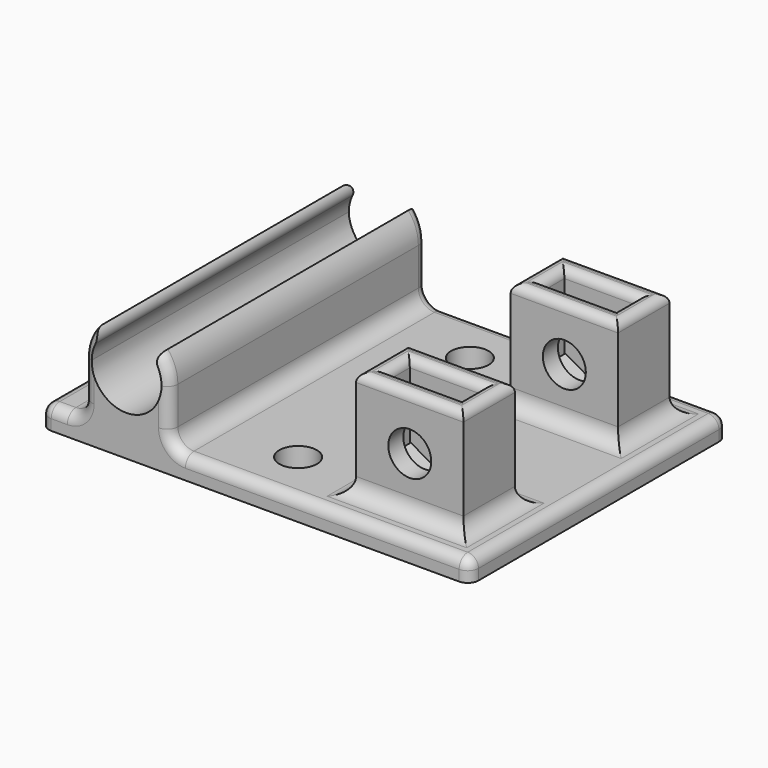
from build123d import *

# Parameters (mm, degrees)
F0_W          = 40
F0_H          = 30
F0_R          = 1.75
F1_DEPTH      = 2
F0_W_2        = 6.8
F0_H_2        = 2.5
F0_W_3        = 10
F0_H_3        = 6
F0_H_4        = 12
F2_DEPTH      = 12
F3_R          = 2
F4_DEPTH      = 24
F5_DEPTH      = 24
F6_START      = 2
F6_DEPTH      = 10
F7_R          = 1.5
F8_R          = 0.79999
F11_DEPTH     = 30
F12_T1_DEPTH  = 33.8160542738
F13_R         = 1.5
F14_T1_DEPTH  = 3.5
F14_T3_DEPTH  = 28
F14_T5_DEPTH  = 1.5
F14_T7_DEPTH  = 25.5
F14_T9_DEPTH  = 3.5
F14_S13_W     = 1
F14_S13_H     = 1
F14_T14_DEPTH = 1
F14_S19_W     = 1
F14_S19_H     = 1
F14_T20_DEPTH = 1
F14_S25_W     = 1
F14_S25_H     = 1
F14_T26_DEPTH = 1
F14_S31_W     = 1
F14_S31_H     = 1
F14_T32_DEPTH = 1
F14_T36_ANGLE = 90
F14_T38_ANGLE = 90
F14_T40_ANGLE = 90
F14_T42_ANGLE = 90
F14_T44_ANGLE = 75.8127030586
F14_T46_ANGLE = 75.8127030586
F14_T48_ANGLE = 75.8127030586
F14_T50_ANGLE = 75.8127030586


# Not quite as in the source:
# - a fillet or chamfer that OpenCascade refuses, or shapes differently, is made with other operations: its cross-section is extruded or revolved along the edge and cut away or added
# - a fillet or chamfer is up to 0.001 mm smaller than in the source, because OpenCascade refuses the exact size


with BuildPart() as f1:
    # F0 (on Top) → F1 (new body)
    with BuildSketch(Plane.XY):
        Rectangle(F0_W, F0_H)
        with Locations((0, -10)):
            Circle(F0_R, mode=Mode.SUBTRACT)
        Polygon((17, -12), (7, -12), (7, -6), (7, 6), (7, 12), (17, 12), (17, 6), (17, -6), align=None, mode=Mode.SUBTRACT)
        with Locations((0, 10)):
            Circle(F0_R, mode=Mode.SUBTRACT)
    extrude(amount=F1_DEPTH)



with BuildPart() as f1b:
    # F0 (on Top) → F1, piece 2 (new body)
    with BuildSketch(Plane.XY):
        with Locations((12, 9)):
            Rectangle(F0_W_2, F0_H_2)
    extrude(amount=F1_DEPTH)


with BuildPart() as f1c:
    # F0 (on Top) → F1, piece 3 (new body)
    with BuildSketch(Plane.XY):
        with Locations((12, -9)):
            Rectangle(F0_W_2, F0_H_2)
    extrude(amount=F1_DEPTH)


with BuildPart() as f1_1:
    add(f1.part)

    add(f1b.part)  # F2 merges F1b

    add(f1c.part)  # F2 merges F1c
    # F0 (on Top) → F2 (join)
    with BuildSketch(Plane.XY):
        with Locations((12, -9)):
            Rectangle(F0_W_3, F0_H_3)
        with Locations((12, -9)):
            Rectangle(F0_W_2, F0_H_2, mode=Mode.SUBTRACT)
        with Locations((12, 9)):
            Rectangle(F0_W_3, F0_H_3)
        with Locations((12, 9)):
            Rectangle(F0_W_2, F0_H_2, mode=Mode.SUBTRACT)
        with Locations((12, 0)):
            Rectangle(F0_W_3, F0_H_4)
    extrude(amount=F2_DEPTH)

    # F3 (on face) → F4 (cut, through all)
    with BuildSketch(Plane.XZ.offset(12)):
        with Locations((12, 7)):
            Circle(F3_R)
    extrude(amount=-F4_DEPTH, mode=Mode.SUBTRACT)

    # F3 (on face) → F5 (join, through all)
    with BuildSketch(Plane.XZ.offset(12)):
        Polygon((15.3, 2), (15.3, 5.0947441117), (12, 3.1894882233), (8.7, 5.0947441117), (8.7, 2), align=None)
    extrude(amount=-F5_DEPTH)

    # F0 (on Top) → F6 (cut)
    with BuildSketch(Plane.XY.offset(F6_START)):
        with Locations((12, 0)):
            Rectangle(F0_W_3, F0_H_4)
    extrude(amount=F6_DEPTH, mode=Mode.SUBTRACT)

    # F7
    f7_edges = [f1_1.edges().sort_by_distance(p)[0] for p in [
        (12, -12, 2),
        (17, -9, 2),
        (12, -6, 2),
        (7, -9, 2),
        (12, 6, 2),
        (7, 9, 2),
        (17, 9, 2),
        (12, 12, 2),
    ]]
    fillet(f7_edges, radius=F7_R)

    # F8 (radius 0.8 in the source; OpenCascade refuses exactly that, so slightly less here)
    f8_edges = [f1_1.edges().sort_by_distance(p)[0] for p in [
        (12, -10.25, 12),
        (8.6, -9, 12),
        (12, -7.75, 12),
        (15.4, -9, 12),
        (17, -9, 12),
        (12, -12, 12),
        (12, -6, 12),
        (7, -9, 12),
        (12, 6, 12),
        (7, 9, 12),
        (12, 12, 12),
        (17, 9, 12),
        (15.4, 9, 12),
        (12, 10.25, 12),
        (12, 7.75, 12),
        (8.6, 9, 12),
    ]]
    fillet(f8_edges, radius=F8_R)

    # F10 (on line) → F11 (join, through all)
    with BuildSketch(Plane(origin=(0, -15, 0), x_dir=(-1, 0, 0), z_dir=(0, 1, 0))):
        with BuildLine():
            Line((8, 2), (16, 2))
            Line((16, 2), (16, 7))
            ThreePointArc((16, 7), (15.7587704831, 8.3680805733), (15.0641777725, 9.5711504387))
            Line((15.0641777725, 9.5711504387), (14.4896444401, 9.0890597315))
            ThreePointArc((14.4896444401, 9.0890597315), (15.0540010176, 8.1115654658), (15.25, 7))
            ThreePointArc((15.25, 7), (10.8884345342, 3.9459989824), (9.5103555599, 9.0890597315))
            Line((9.5103555599, 9.0890597315), (8.9358222275, 9.5711504387))
            ThreePointArc((8.9358222275, 9.5711504387), (8.2412295169, 8.3680805733), (8, 7))
            Line((8, 7), (8, 2))
        make_face()
    extrude(amount=F11_DEPTH)

    # F12: fillet of radius 1 on 2 edges, made by hand

    # F12_s2 → F12_t1 (cut)
    with BuildSketch(Plane.XZ.offset(-16.9080271369)):
        with BuildLine():
            ThreePointArc((-15.0641777725, 9.5711504387), (-14.8125666969, 9.0351734886), (-14.9081851274, 8.4508477746))
            ThreePointArc((-14.9081851274, 8.4508477746), (-14.7177140459, 8.782282347), (-14.4896444401, 9.0890597315))
            Line((-14.4896444401, 9.0890597315), (-15.0641777725, 9.5711504387))
        make_face()
        with BuildLine():
            ThreePointArc((-9.0918148726, 8.4508477746), (-9.1874333031, 9.0351734886), (-8.9358222275, 9.5711504387))
            Line((-8.9358222275, 9.5711504387), (-9.5103555599, 9.0890597315))
            ThreePointArc((-9.5103555599, 9.0890597315), (-9.2822859541, 8.782282347), (-9.0918148726, 8.4508477746))
        make_face()
    extrude(amount=F12_T1_DEPTH, mode=Mode.SUBTRACT)

    # F13
    f13_edges = [f1_1.edges().sort_by_distance(p)[0] for p in [
        (-16, 0, 2),
        (-8, 0, 2),
    ]]
    fillet(f13_edges, radius=F13_R)

    # F14: fillet of radius 1 on 18 edges, made by hand

    # F14_s2 → F14_t1 (cut)
    with BuildSketch(Plane.XY.offset(-2.5)):
        with BuildLine():
            ThreePointArc((-19, -15), (-19.7071067812, -14.7071067812), (-20, -14))
            Line((-20, -14), (-20, -15))
            Line((-20, -15), (-19, -15))
        make_face()
        with BuildLine():
            ThreePointArc((-19, 15), (-19.7071067812, 14.7071067812), (-20, 14))
            Line((-20, 14), (-20, 15))
            Line((-20, 15), (-19, 15))
        make_face()
        with BuildLine():
            ThreePointArc((20, 14), (19.7071067812, 14.7071067812), (19, 15))
            Line((19, 15), (20, 15))
            Line((20, 15), (20, 14))
        make_face()
        with BuildLine():
            ThreePointArc((19, -15), (19.7071067812, -14.7071067812), (20, -14))
            Line((20, -14), (20, -15))
            Line((20, -15), (19, -15))
        make_face()
    extrude(amount=F14_T1_DEPTH, mode=Mode.SUBTRACT)

    # F14_s4 → F14_t3 (cut)
    with BuildSketch(Plane.XZ.offset(-14)):
        with BuildLine():
            ThreePointArc((-20, 1), (-19.7071067812, 1.7071067812), (-19, 2))
            Line((-19, 2), (-20, 2))
            Line((-20, 2), (-20, 1))
        make_face()
        with BuildLine():
            ThreePointArc((19, 2), (19.7071067812, 1.7071067812), (20, 1))
            Line((20, 1), (20, 2))
            Line((20, 2), (19, 2))
        make_face()
    extrude(amount=F14_T3_DEPTH, mode=Mode.SUBTRACT)

    # F14_s6 → F14_t5 (cut)
    with BuildSketch(Plane.YZ.offset(-19)):
        with BuildLine():
            ThreePointArc((15, 1), (14.7071067812, 1.7071067812), (14, 2))
            Line((14, 2), (15, 2))
            Line((15, 2), (15, 1))
        make_face()
        with BuildLine():
            ThreePointArc((-15, 1), (-14.7071067812, 1.7071067812), (-14, 2))
            Line((-14, 2), (-15, 2))
            Line((-15, 2), (-15, 1))
        make_face()
    extrude(amount=F14_T5_DEPTH, mode=Mode.SUBTRACT)

    # F14_s8 → F14_t7 (cut)
    with BuildSketch(Plane.YZ.offset(-6.5)):
        with BuildLine():
            ThreePointArc((14, 2), (14.7071067812, 1.7071067812), (15, 1))
            Line((15, 1), (15, 2))
            Line((15, 2), (14, 2))
        make_face()
        with BuildLine():
            ThreePointArc((-14, 2), (-14.7071067812, 1.7071067812), (-15, 1))
            Line((-15, 1), (-15, 2))
            Line((-15, 2), (-14, 2))
        make_face()
    extrude(amount=F14_T7_DEPTH, mode=Mode.SUBTRACT)

    # F14_s10 → F14_t9 (cut)
    with BuildSketch(Plane.XY.offset(3.5)):
        with BuildLine():
            ThreePointArc((-9, -15), (-8.2928932188, -14.7071067812), (-8, -14))
            Line((-8, -14), (-8, -15))
            Line((-8, -15), (-9, -15))
        make_face()
        with BuildLine():
            ThreePointArc((-15, -15), (-15.7071067812, -14.7071067812), (-16, -14))
            Line((-16, -14), (-16, -15))
            Line((-16, -15), (-15, -15))
        make_face()
        with BuildLine():
            ThreePointArc((-15, 15), (-15.7071067812, 14.7071067812), (-16, 14))
            Line((-16, 14), (-16, 15))
            Line((-16, 15), (-15, 15))
        make_face()
        with BuildLine():
            ThreePointArc((-9, 15), (-8.2928932188, 14.7071067812), (-8, 14))
            Line((-8, 14), (-8, 15))
            Line((-8, 15), (-9, 15))
        make_face()
    extrude(amount=F14_T9_DEPTH, mode=Mode.SUBTRACT)


with BuildPart() as f14_tool12:
    # F14_s13 → F14_t14 (new body)
    with BuildSketch(Plane.XZ.offset(14)):
        with Locations((-19.5, 1.5)):
            Rectangle(F14_S13_W, F14_S13_H)
    extrude(amount=F14_T14_DEPTH)

    # F14_s15 → F14_t16 (revolve, cut)
    with BuildSketch(Plane(origin=(-19, -14, 1), x_dir=(0.7071067812, 0, -0.7071067812), z_dir=(-0.7071067812, 0, -0.7071067812))):
        with BuildLine():
            ThreePointArc((0, -1), (1, 0), (0, 1))
            Line((0, 1), (0, -1))
        make_face()
    revolve(axis=Axis((-19, -14, 1), (0, -1, 0)), mode=Mode.SUBTRACT)


with BuildPart() as f1_2:
    add(f1_1.part)

    # F14_t11: cut F14_tool12
    add(f14_tool12.part, mode=Mode.SUBTRACT)


with BuildPart() as f14_tool18:
    # F14_s19 → F14_t20 (new body)
    with BuildSketch(Plane.YZ.offset(-19)):
        with Locations((14.5, 1.5)):
            Rectangle(F14_S19_W, F14_S19_H)
    extrude(amount=-F14_T20_DEPTH)

    # F14_s21 → F14_t22 (revolve, cut)
    with BuildSketch(Plane(origin=(-19, 14, 1), x_dir=(0, -0.7071067812, -0.7071067812), z_dir=(0, 0.7071067812, -0.7071067812))):
        with BuildLine():
            ThreePointArc((0, -1), (1, 0), (0, 1))
            Line((0, 1), (0, -1))
        make_face()
    revolve(axis=Axis((-19, 14, 1), (-1, 0, 0)), mode=Mode.SUBTRACT)


with BuildPart() as f1_3:
    add(f1_2.part)

    # F14_t17: cut F14_tool18
    add(f14_tool18.part, mode=Mode.SUBTRACT)


with BuildPart() as f14_tool24:
    # F14_s25 → F14_t26 (new body)
    with BuildSketch(Plane.XY.offset(1)):
        with Locations((19.5, 14.5)):
            Rectangle(F14_S25_W, F14_S25_H)
    extrude(amount=F14_T26_DEPTH)

    # F14_s27 → F14_t28 (revolve, cut)
    with BuildSketch(Plane(origin=(19, 14, 1), x_dir=(-0.7071067812, -0.7071067812, 0), z_dir=(-0.7071067812, 0.7071067812, 0))):
        with BuildLine():
            ThreePointArc((0, -1), (1, 0), (0, 1))
            Line((0, 1), (0, -1))
        make_face()
    revolve(axis=Axis((19, 14, 1), (0, 0, 1)), mode=Mode.SUBTRACT)


with BuildPart() as f1_4:
    add(f1_3.part)

    # F14_t23: cut F14_tool24
    add(f14_tool24.part, mode=Mode.SUBTRACT)


with BuildPart() as f14_tool30:
    # F14_s31 → F14_t32 (new body)
    with BuildSketch(Plane.XY.offset(1)):
        with Locations((19.5, -14.5)):
            Rectangle(F14_S31_W, F14_S31_H)
    extrude(amount=F14_T32_DEPTH)

    # F14_s33 → F14_t34 (revolve, cut)
    with BuildSketch(Plane(origin=(19, -14, 1), x_dir=(-0.7071067812, 0.7071067812, 0), z_dir=(0.7071067812, 0.7071067812, 0))):
        with BuildLine():
            ThreePointArc((0, -1), (1, 0), (0, 1))
            Line((0, 1), (0, -1))
        make_face()
    revolve(axis=Axis((19, -14, 1), (0, 0, 1)), mode=Mode.SUBTRACT)


with BuildPart() as f1_5:
    add(f1_4.part)

    # F14_t29: cut F14_tool30
    add(f14_tool30.part, mode=Mode.SUBTRACT)

    # F14_s35 → F14_t36 (revolve, cut)
    with BuildSketch(Plane.YZ.offset(-6.5)):
        with BuildLine():
            ThreePointArc((-15, 1), (-14.7071067812, 1.7071067812), (-14, 2))
            Line((-14, 2), (-15, 2))
            Line((-15, 2), (-15, 1))
        make_face()
    revolve(axis=Axis((-6.5, -15, 3.5), (0, 1, 0)), revolution_arc=F14_T36_ANGLE, mode=Mode.SUBTRACT)

    # F14_s37 → F14_t38 (revolve, cut)
    with BuildSketch(Plane.XY.offset(3.5)):
        with BuildLine():
            ThreePointArc((-15, -15), (-15.7071067812, -14.7071067812), (-16, -14))
            Line((-16, -14), (-16, -15))
            Line((-16, -15), (-15, -15))
        make_face()
    revolve(axis=Axis((-17.5, -15, 3.5), (0, 1, 0)), revolution_arc=F14_T38_ANGLE, mode=Mode.SUBTRACT)

    # F14_s39 → F14_t40 (revolve, cut)
    with BuildSketch(Plane.YZ.offset(-6.5)):
        with BuildLine():
            ThreePointArc((14, 2), (14.7071067812, 1.7071067812), (15, 1))
            Line((15, 1), (15, 2))
            Line((15, 2), (14, 2))
        make_face()
    revolve(axis=Axis((-6.5, 15, 3.5), (0, 1, 0)), revolution_arc=F14_T40_ANGLE, mode=Mode.SUBTRACT)

    # F14_s41 → F14_t42 (revolve, cut)
    with BuildSketch(Plane.XY.offset(3.5)):
        with BuildLine():
            ThreePointArc((-15, 15), (-15.7071067812, 14.7071067812), (-16, 14))
            Line((-16, 14), (-16, 15))
            Line((-16, 15), (-15, 15))
        make_face()
    revolve(axis=Axis((-17.5, 15, 3.5), (0, 1, 0)), revolution_arc=F14_T42_ANGLE, mode=Mode.SUBTRACT)

    # F14_s43 → F14_t44 (revolve, cut)
    with BuildSketch(Plane(origin=(-12.9424757059, 0, 3.2718967917), x_dir=(0, 1, 0), z_dir=(-0.9694997132, 0, 0.2450924439))):
        with BuildLine():
            ThreePointArc((15, -6.8453886653), (14.7071067812, -7.5524954465), (14, -7.8453886653))
            Line((14, -7.8453886653), (15, -7.8453886653))
            Line((15, -7.8453886653), (15, -6.8453886653))
        make_face()
    revolve(axis=Axis((-12, 15, 7), (0, 1, 0)), revolution_arc=F14_T44_ANGLE, mode=Mode.SUBTRACT)

    # F14_s45 → F14_t46 (revolve, cut)
    with BuildSketch(Plane.XY.offset(7)):
        with BuildLine():
            ThreePointArc((-15, 15), (-15.7071067812, 14.7071067812), (-16, 14))
            Line((-16, 14), (-16, 15))
            Line((-16, 15), (-15, 15))
        make_face()
    revolve(axis=Axis((-12, 15, 7), (0, 1, 0)), revolution_arc=F14_T46_ANGLE, mode=Mode.SUBTRACT)

    # F14_s47 → F14_t48 (revolve, cut)
    with BuildSketch(Plane.XY.offset(7)):
        with BuildLine():
            ThreePointArc((-15, -15), (-15.7071067812, -14.7071067812), (-16, -14))
            Line((-16, -14), (-16, -15))
            Line((-16, -15), (-15, -15))
        make_face()
    revolve(axis=Axis((-12, -15, 7), (0, 1, 0)), revolution_arc=F14_T48_ANGLE, mode=Mode.SUBTRACT)

    # F14_s49 → F14_t50 (revolve, cut)
    with BuildSketch(Plane(origin=(-12.9424757059, 0, 3.2718967917), x_dir=(0, 1, 0), z_dir=(-0.9694997132, 0, 0.2450924439))):
        with BuildLine():
            ThreePointArc((-15, -6.8453886653), (-14.7071067812, -7.5524954465), (-14, -7.8453886653))
            Line((-14, -7.8453886653), (-15, -7.8453886653))
            Line((-15, -7.8453886653), (-15, -6.8453886653))
        make_face()
    revolve(axis=Axis((-12, -15, 7), (0, 1, 0)), revolution_arc=F14_T50_ANGLE, mode=Mode.SUBTRACT)


solid = f1_5.part
